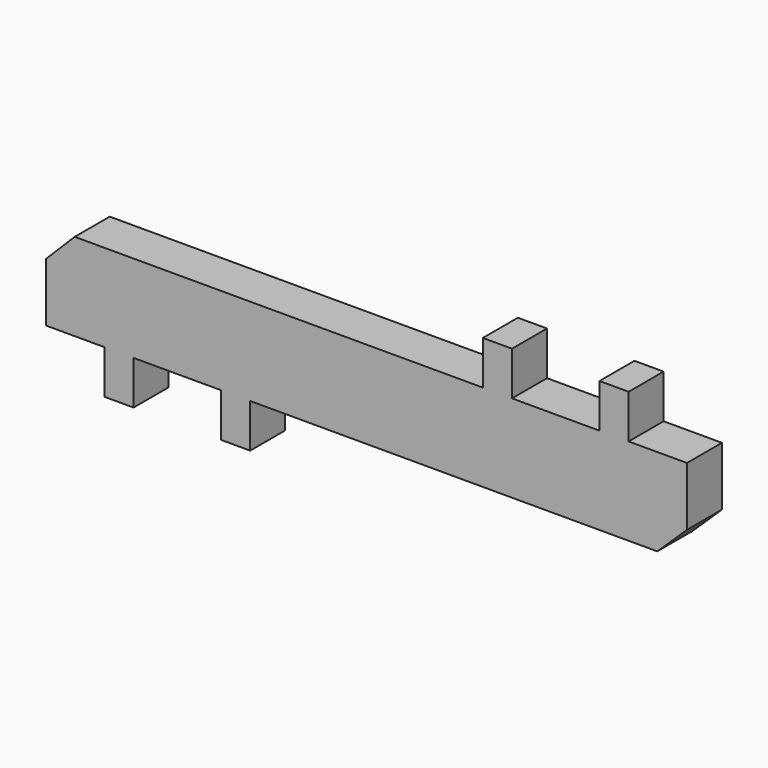
from build123d import *

# Parameters (mm, degrees)
F1_DEPTH = 19.05


# Not quite as in the source:
# - a feature names something its author has since deleted; it is built from what else it names


with BuildPart() as f1:
    # F0 (on Front) → F1 (new body)
    with BuildSketch(Plane.XZ):
        Polygon((-140.5185023113, -17.3581795608), (-115.1141719677, -17.3581795608), (-115.1141719677, -36.4081795608), (-102.4141719677, -36.4081795608), (-102.4141719677, -17.3581795608), (-64.3141719677, -17.3581795608), (-64.3141719677, -36.4081795608), (-51.6141719677, -36.4081795608), (-51.6141719677, -17.3581795608), (125.7340388179, -17.3581795608), (138.656257718, -4.8882621778), (138.656257718, 20.7418204392), (113.256257718, 20.7418204392), (113.256257718, 39.7918204392), (100.556257718, 39.7918204392), (100.556257718, 20.7418204392), (62.456257718, 20.7418204392), (62.456257718, 39.7918204392), (49.756257718, 39.7918204392), (49.756257718, 20.7418204392), (-128.043742282, 20.7418204392), (-140.5185023113, 8.2640567404), align=None)
    extrude(amount=F1_DEPTH)


solid = f1.part
